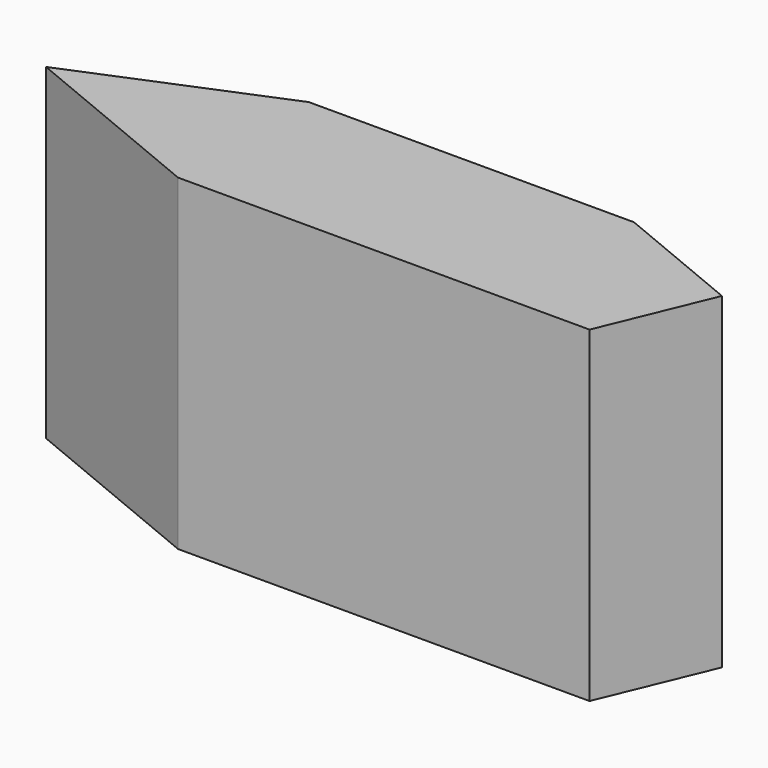
from build123d import *

# Parameters (mm, degrees)
F0_W          = 6.35
F0_H          = 12.7
F1_DEPTH      = 12.7
F3_DEPTH      = 6.351
F3_DEPTH_BACK = 6.351
F5_DEPTH      = 6.351
F5_DEPTH_BACK = 6.351
F7_DEPTH      = 6.351
F7_DEPTH_BACK = 6.351


# Not quite as in the source:
# - a pattern or mirror of a feature is missing from the dataset's text; its kind, count and spacing are read off the source's solid


with BuildPart() as f1:
    # F0 (on Right) → F1 (new body, symmetric)
    with BuildSketch(Plane.YZ):
        Rectangle(F0_W, F0_H)
    extrude(amount=F1_DEPTH, both=True)

    # F2 (on Top) → F3 (cut, two sides)
    with BuildSketch(Plane.XY) as f3_sk:
        Polygon((-12.7, 3.175), (-12.7, 0), (-5.0348719395, 3.175), align=None)
    f3 = extrude(amount=-F3_DEPTH, mode=Mode.SUBTRACT) + extrude(f3_sk.sketch, amount=F3_DEPTH_BACK, mode=Mode.SUBTRACT)

    # F3_copies: F3 across plane
    add(f3.mirror(Plane(origin=(0, 0, 0), x_dir=(0, 0, -1), z_dir=(0, -1, 0))), mode=Mode.SUBTRACT)

    # F4 (on Top) → F5 (cut, two sides)
    with BuildSketch(Plane.XY) as f5_sk:
        Polygon((17.9670583457, 3.175), (7.5919586605, 3.175), (12.7, 1.05918), align=None)
    extrude(amount=-F5_DEPTH, mode=Mode.SUBTRACT)
    extrude(f5_sk.sketch, amount=F5_DEPTH_BACK, mode=Mode.SUBTRACT)

    # F6 (on Top) → F7 (cut, two sides)
    with BuildSketch(Plane.XY) as f7_sk:
        Polygon((12.7, 1.05918), (10.9461452185, -3.175), (12.7, -3.175), align=None)
    extrude(amount=-F7_DEPTH, mode=Mode.SUBTRACT)
    extrude(f7_sk.sketch, amount=F7_DEPTH_BACK, mode=Mode.SUBTRACT)


solid = f1.part
